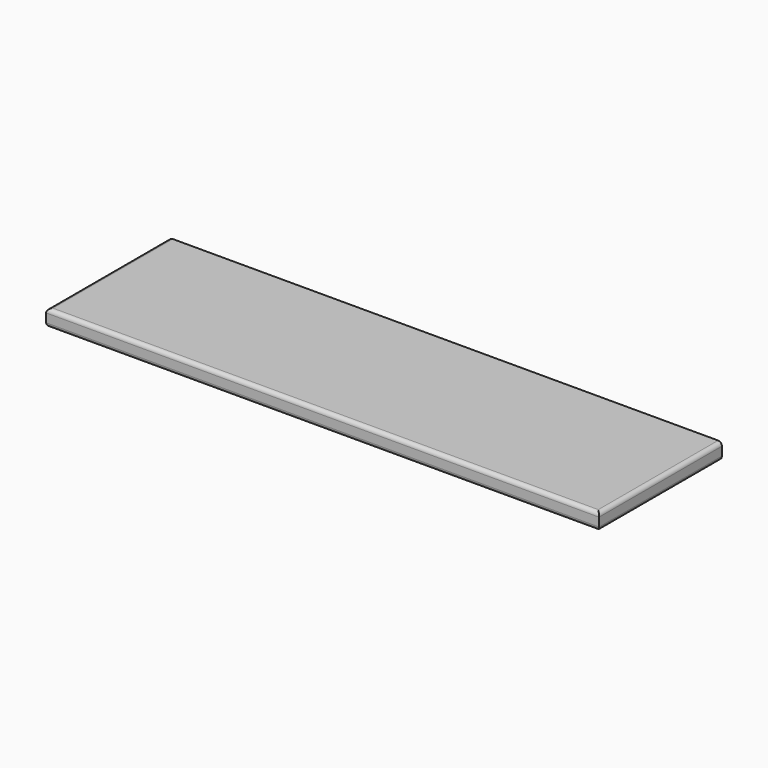
from build123d import *

# Parameters (mm, degrees)
F0_W        = 914.4
F0_H        = 254
F1_DEPTH    = 26.9875
F2_R        = 6.35
F3_T1_DEPTH = 279.4
F4_T1_DEPTH = 279.4


# Not quite as in the source:
# - a fillet or chamfer that OpenCascade refuses, or shapes differently, is made with other operations: its cross-section is extruded or revolved along the edge and cut away or added


with BuildPart() as f1:
    # F0 (on Top) → F1 (new body)
    with BuildSketch(Plane.XY):
        with Locations((0, 101.6)):
            Rectangle(F0_W, F0_H)
    extrude(amount=F1_DEPTH)

    # F2
    f2_edges = [f1.edges().sort_by_distance(p)[0] for p in [
        (0, -25.4, 26.9875),
        (0, -25.4, 0),
    ]]
    fillet(f2_edges, radius=F2_R)

    # F3: fillet of radius 6.35 on 2 edges, made by hand

    # F3_s2 → F3_t1 (cut)
    with BuildSketch(Plane.XZ.offset(-244.475)):
        with BuildLine():
            ThreePointArc((450.85, 26.9875), (455.3401280605, 25.1276280605), (457.2, 20.6375))
            Line((457.2, 20.6375), (457.2, 26.9875))
            Line((457.2, 26.9875), (450.85, 26.9875))
        make_face()
        with BuildLine():
            ThreePointArc((450.85, 0), (455.3401280605, 1.8598719395), (457.2, 6.35))
            Line((457.2, 6.35), (457.2, 0))
            Line((457.2, 0), (450.85, 0))
        make_face()
    extrude(amount=F3_T1_DEPTH, mode=Mode.SUBTRACT)

    # F4: fillet of radius 6.35 on 2 edges, made by hand

    # F4_s2 → F4_t1 (cut)
    with BuildSketch(Plane.XZ.offset(-244.475)):
        with BuildLine():
            ThreePointArc((-457.2, 6.35), (-455.3401280605, 1.8598719395), (-450.85, 0))
            Line((-450.85, 0), (-457.2, 0))
            Line((-457.2, 0), (-457.2, 6.35))
        make_face()
        with BuildLine():
            ThreePointArc((-457.2, 20.6375), (-455.3401280605, 25.1276280605), (-450.85, 26.9875))
            Line((-450.85, 26.9875), (-457.2, 26.9875))
            Line((-457.2, 26.9875), (-457.2, 20.6375))
        make_face()
    extrude(amount=F4_T1_DEPTH, mode=Mode.SUBTRACT)


solid = f1.part
